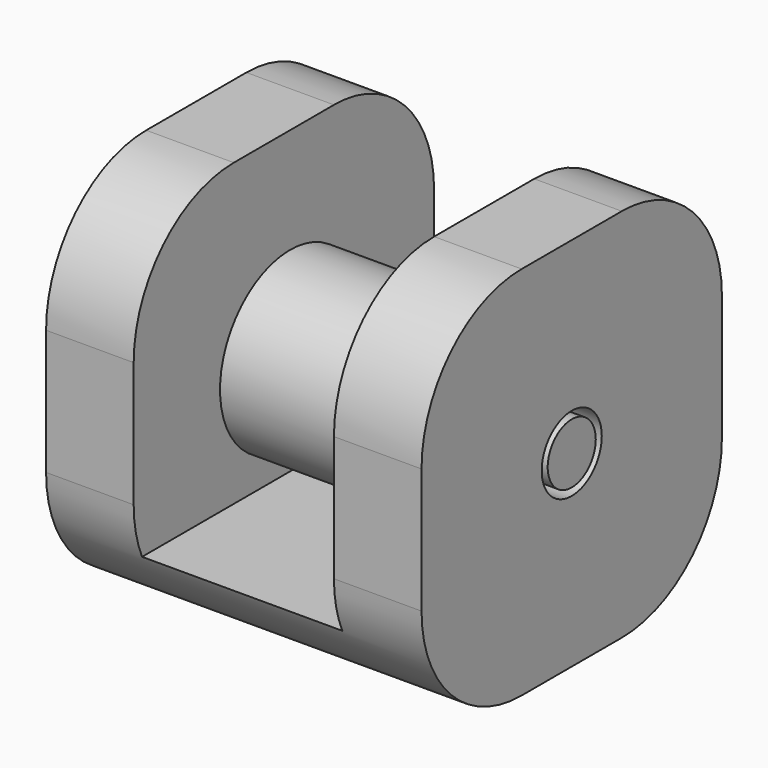
from build123d import *

# Parameters (mm, degrees)
F0_W         = 15
F0_H         = 15
F1_DEPTH     = 15
F3_D         = 3
F4_W         = 8
F4_H         = 12
F5_DEPTH     = 15.001
F6_R         = 3.5
F7_DEPTH     = 3.75
F8_R         = 1.2
F9_DEPTH     = 3.75
F10_T1_DEPTH = 28.5
F10_T3_DEPTH = 28.5
F10_T5_DEPTH = 40


# Not quite as in the source:
# - a fillet or chamfer that OpenCascade refuses, or shapes differently, is made with other operations: its cross-section is extruded or revolved along the edge and cut away or added
# - a pattern or mirror of a feature is missing from the dataset's text; its kind, count and spacing are read off the source's solid


with BuildPart() as f1:
    # F0 (on Top) → F1 (new body)
    with BuildSketch(Plane.XY):
        Rectangle(F0_W, F0_H)
    extrude(amount=F1_DEPTH)

    # F3 (through all)
    with Locations(Plane(origin=(-7.5, 0, 0), x_dir=(0, -1, 0), z_dir=(-1, 0, 0))):
        with Locations((0, 7.5)):
            Hole(F3_D / 2)

    # F4 (on face) → F5 (cut, through all)
    with BuildSketch(Plane(origin=(0, 7.5, 0), x_dir=(-1, 0, 0), z_dir=(0, 1, 0))):
        with Locations((0, 9)):
            Rectangle(F4_W, F4_H)
    extrude(amount=-F5_DEPTH, mode=Mode.SUBTRACT)

    # F10: fillet of radius 5 on 6 edges, made by hand

    # F10_s2 → F10_t1 (cut)
    with BuildSketch(Plane.YZ.offset(-20)):
        with BuildLine():
            ThreePointArc((-7.5, 10), (-6.0355339059, 13.5355339059), (-2.5, 15))
            Line((-2.5, 15), (-7.5, 15))
            Line((-7.5, 15), (-7.5, 10))
        make_face()
        with BuildLine():
            ThreePointArc((7.5, 10), (6.0355339059, 13.5355339059), (2.5, 15))
            Line((2.5, 15), (7.5, 15))
            Line((7.5, 15), (7.5, 10))
        make_face()
    extrude(amount=F10_T1_DEPTH, mode=Mode.SUBTRACT)

    # F10_s4 → F10_t3 (cut)
    with BuildSketch(Plane.YZ.offset(-8.5)):
        with BuildLine():
            ThreePointArc((-7.5, 10), (-6.0355339059, 13.5355339059), (-2.5, 15))
            Line((-2.5, 15), (-7.5, 15))
            Line((-7.5, 15), (-7.5, 10))
        make_face()
        with BuildLine():
            ThreePointArc((2.5, 15), (6.0355339059, 13.5355339059), (7.5, 10))
            Line((7.5, 10), (7.5, 15))
            Line((7.5, 15), (2.5, 15))
        make_face()
    extrude(amount=F10_T3_DEPTH, mode=Mode.SUBTRACT)

    # F10_s6 → F10_t5 (cut)
    with BuildSketch(Plane.YZ.offset(-20)):
        with BuildLine():
            ThreePointArc((2.5, 0), (6.0355339059, 1.4644660941), (7.5, 5))
            Line((7.5, 5), (7.5, 0))
            Line((7.5, 0), (2.5, 0))
        make_face()
        with BuildLine():
            ThreePointArc((-7.5, 5), (-6.0355339059, 1.4644660941), (-2.5, 0))
            Line((-2.5, 0), (-7.5, 0))
            Line((-7.5, 0), (-7.5, 5))
        make_face()
    extrude(amount=F10_T5_DEPTH, mode=Mode.SUBTRACT)


with BuildPart() as f7:
    # F6 (on Right) → F7 (new body, symmetric)
    with BuildSketch(Plane.YZ):
        with Locations((0, 7.5)):
            Circle(F6_R)
    extrude(amount=F7_DEPTH, both=True)

    # F8 (on face) → F9 (join)
    with BuildSketch(Plane.YZ.offset(3.75)):
        with Locations((0, 7.5)):
            Circle(F8_R)
    f9 = extrude(amount=F9_DEPTH)

    # F9_copies: F9 across plane
    add(f9.mirror(Plane(origin=(0, 0, 0), x_dir=(0, 0, -1), z_dir=(-1, 0, 0))))


solid = Compound([f1.part, f7.part])
